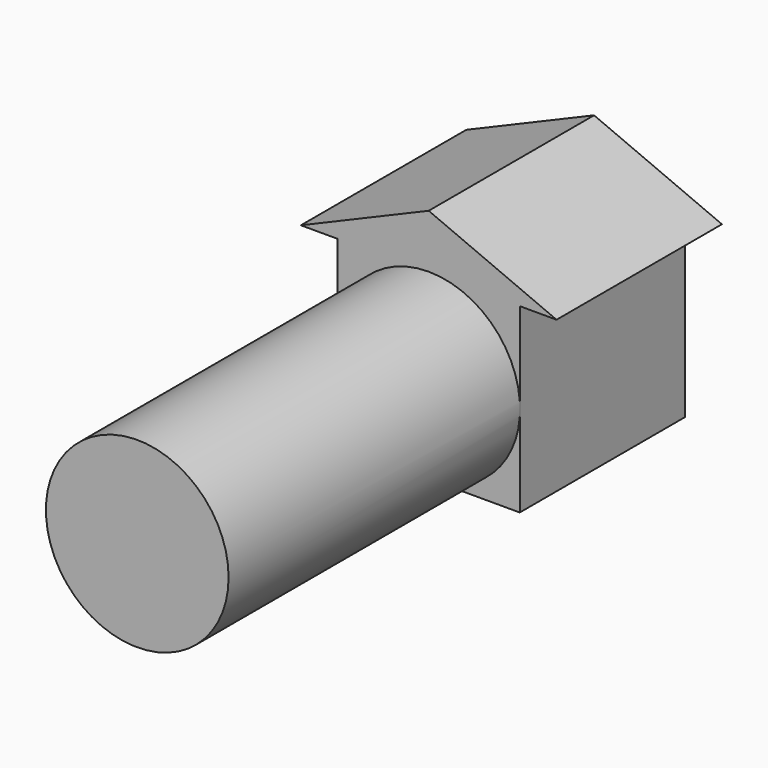
from build123d import *

# Parameters (mm, degrees)
F0_R     = 25.4758585114
F1_DEPTH = 101.6
F3_W     = 50.8
F3_H     = 50.8
F4_DEPTH = 57.658
F6_DEPTH = 57.658


# Not quite as in the source:
# - the program builds the solid bodies; features that only make, move or delete a surface that nothing else refers to are left out


with BuildPart() as f1:
    # F0 (on Front) → F1 (new body)
    with BuildSketch(Plane.XZ):
        Circle(F0_R)
    extrude(amount=F1_DEPTH)

    # F3 (on Front) → F4 (join)
    with BuildSketch(Plane.XZ):
        Rectangle(F3_W, F3_H)
    extrude(amount=-F4_DEPTH)

    # F5 (on Front) → F6 (join)
    with BuildSketch(Plane.XZ):
        Polygon((35.6535799801, 25.266315788), (0, 40.4261052608), (-35.6535799801, 25.266315788), align=None)
    extrude(amount=-F6_DEPTH)


solid = f1.part
